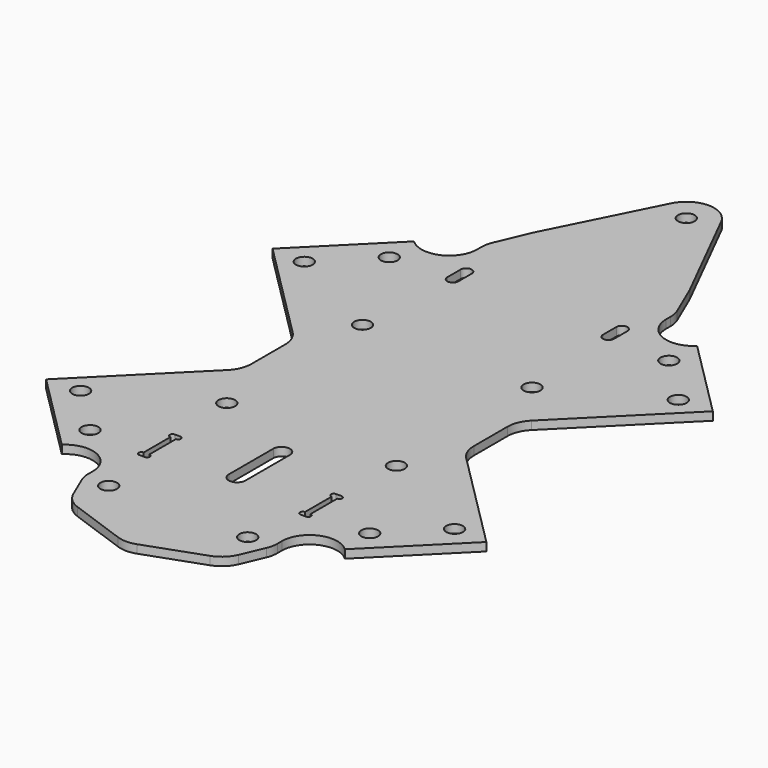
from build123d import *

# Parameters (mm, degrees)
F0_R        = 1.5
F1_DEPTH    = 1.5
F2_T1_DEPTH = 1.5
F3_T1_DEPTH = 1.5
F3_T3_DEPTH = 6.6314425489
F3_T5_DEPTH = 12.4086164325
F3_T7_DEPTH = 10.4285714286
F3_T9_DEPTH = 2.253003807
F5_DEPTH    = 25


# Not quite as in the source:
# - a fillet or chamfer that OpenCascade refuses, or shapes differently, is made with other operations: its cross-section is extruded or revolved along the edge and cut away or added


with BuildPart() as f1:
    # F0 (on Top) → F1 (new body)
    with BuildSketch(Plane.XY):
        with BuildLine():
            Line((-25.4558441227, 39.5979797464), (-39.5979797464, 25.4558441227))
            Line((-39.5979797464, 25.4558441227), (-20, 5.8578643763))
            Line((-20, 5.8578643763), (-20, -5.8578643763))
            Line((-20, -5.8578643763), (-39.5979797464, -25.4558441227))
            Line((-39.5979797464, -25.4558441227), (-25.4558441227, -39.5979797464))
            Line((-25.4558441227, -39.5979797464), (-17, -31.1421356237))
            Line((-17, -31.1421356237), (-17, -45.25))
            Line((-17, -45.25), (-14, -52.25))
            Line((-14, -52.25), (0, -57.25))
            Line((0, -57.25), (14, -52.25))
            Line((14, -52.25), (17, -45.25))
            Line((17, -45.25), (17, -31.1421356237))
            Line((17, -31.1421356237), (25.4558441227, -39.5979797464))
            Line((25.4558441227, -39.5979797464), (39.5979797464, -25.4558441227))
            Line((39.5979797464, -25.4558441227), (20, -5.8578643763))
            Line((20, -5.8578643763), (20, 5.8578643763))
            Line((20, 5.8578643763), (39.5979797464, 25.4558441227))
            Line((39.5979797464, 25.4558441227), (25.4558441227, 39.5979797464))
            Line((25.4558441227, 39.5979797464), (17, 31.1421356237))
            Line((17, 31.1421356237), (17, 45.25))
            Line((17, 45.25), (14, 52.25))
            Line((14, 52.25), (4.468852459, 71.2426229508))
            ThreePointArc((4.468852459, 71.2426229508), (0, 74), (-4.468852459, 71.2426229508))
            Line((-4.468852459, 71.2426229508), (-14, 52.25))
            Line((-14, 52.25), (-17, 45.25))
            Line((-17, 45.25), (-17, 31.1421356237))
            Line((-17, 31.1421356237), (-25.4558441227, 39.5979797464))
        make_face()
        with Locations((-33.6347763109, -25.1494949366)):
            Circle(F0_R, mode=Mode.SUBTRACT)
        with Locations((-25.1494949366, -33.6347763109)):
            Circle(F0_R, mode=Mode.SUBTRACT)
        with Locations((-12.5, -45.25)):
            Circle(F0_R, mode=Mode.SUBTRACT)
        with BuildLine():
            ThreePointArc((-1.5, -22), (0, -20.5), (1.5, -22))
            Line((1.5, -22), (1.5, -32))
            ThreePointArc((1.5, -32), (0, -33.5), (-1.5, -32))
            Line((-1.5, -32), (-1.5, -22))
        make_face(mode=Mode.SUBTRACT)
        with Locations((-15.25, -15.25)):
            Circle(F0_R, mode=Mode.SUBTRACT)
        with Locations((12.5, -45.25)):
            Circle(F0_R, mode=Mode.SUBTRACT)
        with Locations((25.1494949366, -33.6347763109)):
            Circle(F0_R, mode=Mode.SUBTRACT)
        with Locations((33.6347763109, -25.1494949366)):
            Circle(F0_R, mode=Mode.SUBTRACT)
        with Locations((15.25, -15.25)):
            Circle(F0_R, mode=Mode.SUBTRACT)
        with Locations((-33.6347763109, 25.1494949366)):
            Circle(F0_R, mode=Mode.SUBTRACT)
        with Locations((-25.1494949366, 33.6347763109)):
            Circle(F0_R, mode=Mode.SUBTRACT)
        with Locations((-15.25, 15.25)):
            Circle(F0_R, mode=Mode.SUBTRACT)
        with BuildLine():
            Line((-15, 34), (-15, 37))
            ThreePointArc((-15, 37), (-14, 38), (-13, 37))
            Line((-13, 37), (-13, 34))
            ThreePointArc((-13, 34), (-14, 33), (-15, 34))
        make_face(mode=Mode.SUBTRACT)
        with Locations((0, 69)):
            Circle(F0_R, mode=Mode.SUBTRACT)
        with Locations((15.25, 15.25)):
            Circle(F0_R, mode=Mode.SUBTRACT)
        with BuildLine():
            ThreePointArc((13, 37), (14, 38), (15, 37))
            Line((15, 37), (15, 34))
            ThreePointArc((15, 34), (14, 33), (13, 34))
            Line((13, 34), (13, 37))
        make_face(mode=Mode.SUBTRACT)
        with Locations((25.1494949366, 33.6347763109)):
            Circle(F0_R, mode=Mode.SUBTRACT)
        with Locations((33.6347763109, 25.1494949366)):
            Circle(F0_R, mode=Mode.SUBTRACT)
    extrude(amount=F1_DEPTH)

    # F2: fillet of radius 5 on 4 edges, made by hand

    # F2_s2 → F2_t1 (join)
    with BuildSketch(Plane.XY):
        with BuildLine():
            ThreePointArc((17, -43.2114464198), (20.0352125578, -38.613663225), (25.4558441227, -39.5979797464))
            Line((25.4558441227, -39.5979797464), (17, -31.1421356237))
            Line((17, -31.1421356237), (17, -43.2114464198))
        make_face()
        with BuildLine():
            ThreePointArc((-25.4558441227, -39.5979797464), (-20.0352125578, -38.613663225), (-17, -43.2114464198))
            Line((-17, -43.2114464198), (-17, -31.1421356237))
            Line((-17, -31.1421356237), (-25.4558441227, -39.5979797464))
        make_face()
        with BuildLine():
            ThreePointArc((-17, 43.2114464198), (-20.0352125578, 38.613663225), (-25.4558441227, 39.5979797464))
            Line((-25.4558441227, 39.5979797464), (-17, 31.1421356237))
            Line((-17, 31.1421356237), (-17, 43.2114464198))
        make_face()
        with BuildLine():
            ThreePointArc((25.4558441227, 39.5979797464), (20.0352125578, 38.613663225), (17, 43.2114464198))
            Line((17, 43.2114464198), (17, 31.1421356237))
            Line((17, 31.1421356237), (25.4558441227, 39.5979797464))
        make_face()
    extrude(amount=F2_T1_DEPTH)

    # F3: fillet of radius 5 on 13 edges, made by hand

    # F3_s2 → F3_t1 (join)
    with BuildSketch(Plane.XY):
        with BuildLine():
            ThreePointArc((20, 3.7867965644), (20.3806023374, 5.7002137262), (21.4644660941, 7.3223304703))
            Line((21.4644660941, 7.3223304703), (20, 5.8578643763))
            Line((20, 5.8578643763), (20, 3.7867965644))
        make_face()
        with BuildLine():
            ThreePointArc((21.4644660941, -7.3223304703), (20.3806023374, -5.7002137262), (20, -3.7867965644))
            Line((20, -3.7867965644), (20, -5.8578643763))
            Line((20, -5.8578643763), (21.4644660941, -7.3223304703))
        make_face()
        with BuildLine():
            ThreePointArc((-20, -3.7867965644), (-20.3806023374, -5.7002137262), (-21.4644660941, -7.3223304703))
            Line((-21.4644660941, -7.3223304703), (-20, -5.8578643763))
            Line((-20, -5.8578643763), (-20, -3.7867965644))
        make_face()
        with BuildLine():
            ThreePointArc((-21.4644660941, 7.3223304703), (-20.3806023374, 5.7002137262), (-20, 3.7867965644))
            Line((-20, 3.7867965644), (-20, 5.8578643763))
            Line((-20, 5.8578643763), (-21.4644660941, 7.3223304703))
        make_face()
    extrude(amount=F3_T1_DEPTH)

    # F3_s4 → F3_t3 (cut)
    with BuildSketch(Plane.XY.offset(-2.5657212744)):
        with BuildLine():
            ThreePointArc((16.5957251501, -46.1933079831), (16.897888614, -45.2290408516), (17, -44.2237114902))
            Line((17, -44.2237114902), (17, -45.25))
            Line((17, -45.25), (16.5957251501, -46.1933079831))
        make_face()
        with BuildLine():
            ThreePointArc((-17, -44.2237114902), (-16.897888614, -45.2290408516), (-16.5957251501, -46.1933079831))
            Line((-16.5957251501, -46.1933079831), (-17, -45.25))
            Line((-17, -45.25), (-17, -44.2237114902))
        make_face()
        with BuildLine():
            ThreePointArc((-17, 44.2237114902), (-16.897888614, 45.2290408516), (-16.5957251501, 46.1933079831))
            Line((-16.5957251501, 46.1933079831), (-17, 45.25))
            Line((-17, 45.25), (-17, 44.2237114902))
        make_face()
        with BuildLine():
            ThreePointArc((17, 44.2237114902), (16.897888614, 45.2290408516), (16.5957251501, 46.1933079831))
            Line((16.5957251501, 46.1933079831), (17, 45.25))
            Line((17, 45.25), (17, 44.2237114902))
        make_face()
    extrude(amount=F3_T3_DEPTH, mode=Mode.SUBTRACT)

    # F3_s6 → F3_t5 (cut)
    with BuildSketch(Plane.XY.offset(-5.4543082162)):
        with BuildLine():
            ThreePointArc((11.9453797416, -52.9837929494), (13.6881897161, -51.9182763344), (14.8594229067, -50.2446798843))
            Line((14.8594229067, -50.2446798843), (14, -52.25))
            Line((14, -52.25), (11.9453797416, -52.9837929494))
        make_face()
        with BuildLine():
            ThreePointArc((-14.8594229067, -50.2446798843), (-13.6881897161, -51.9182763344), (-11.9453797416, -52.9837929494))
            Line((-11.9453797416, -52.9837929494), (-14, -52.25))
            Line((-14, -52.25), (-14.8594229067, -50.2446798843))
        make_face()
    extrude(amount=F3_T5_DEPTH, mode=Mode.SUBTRACT)

    # F3_s8 → F3_t7 (cut)
    with BuildSketch(Plane.XY.offset(-4.4642857143)):
        with BuildLine():
            ThreePointArc((-1.681681985, -56.6493992911), (0, -56.9406897331), (1.681681985, -56.6493992911))
            Line((1.681681985, -56.6493992911), (0, -57.25))
            Line((0, -57.25), (-1.681681985, -56.6493992911))
        make_face()
    extrude(amount=F3_T7_DEPTH, mode=Mode.SUBTRACT)

    # F3_s10 → F3_t9 (cut)
    with BuildSketch(Plane.XY.offset(-0.3765019035)):
        with BuildLine():
            ThreePointArc((-13.9324518552, 52.3846025166), (-13.9979436343, 52.2490444272), (-14.0593245463, 52.1115760587))
            Line((-14.0593245463, 52.1115760587), (-14, 52.25))
            Line((-14, 52.25), (-13.9324518552, 52.3846025166))
        make_face()
        with BuildLine():
            ThreePointArc((14.0593245463, 52.1115760587), (13.9979436343, 52.2490444272), (13.9324518552, 52.3846025166))
            Line((13.9324518552, 52.3846025166), (14, 52.25))
            Line((14, 52.25), (14.0593245463, 52.1115760587))
        make_face()
    extrude(amount=F3_T9_DEPTH, mode=Mode.SUBTRACT)

    # F4 (on face) → F5 (cut)
    with BuildSketch(Plane.XY.offset(1.5)):
        with BuildLine():
            Line((-14, -27.25), (-15, -27.25))
            ThreePointArc((-15, -27.25), (-15.5, -27.75), (-15, -28.25))
            Line((-15, -28.25), (-15, -34.25))
            ThreePointArc((-15, -34.25), (-15.5, -34.75), (-15, -35.25))
            Line((-15, -35.25), (-14, -35.25))
            ThreePointArc((-14, -35.25), (-13.5, -34.75), (-14, -34.25))
            Line((-14, -34.25), (-14, -28.25))
            ThreePointArc((-14, -28.25), (-13.5, -27.75), (-14, -27.25))
        make_face()
        with BuildLine():
            ThreePointArc((15, -28.25), (15.5, -27.75), (15, -27.25))
            Line((15, -27.25), (14, -27.25))
            ThreePointArc((14, -27.25), (13.5, -27.75), (14, -28.25))
            Line((14, -28.25), (14, -34.25))
            ThreePointArc((14, -34.25), (13.5, -34.75), (14, -35.25))
            Line((14, -35.25), (15, -35.25))
            ThreePointArc((15, -35.25), (15.5, -34.75), (15, -34.25))
            Line((15, -34.25), (15, -28.25))
        make_face()
    extrude(amount=-F5_DEPTH, mode=Mode.SUBTRACT)


solid = f1.part
